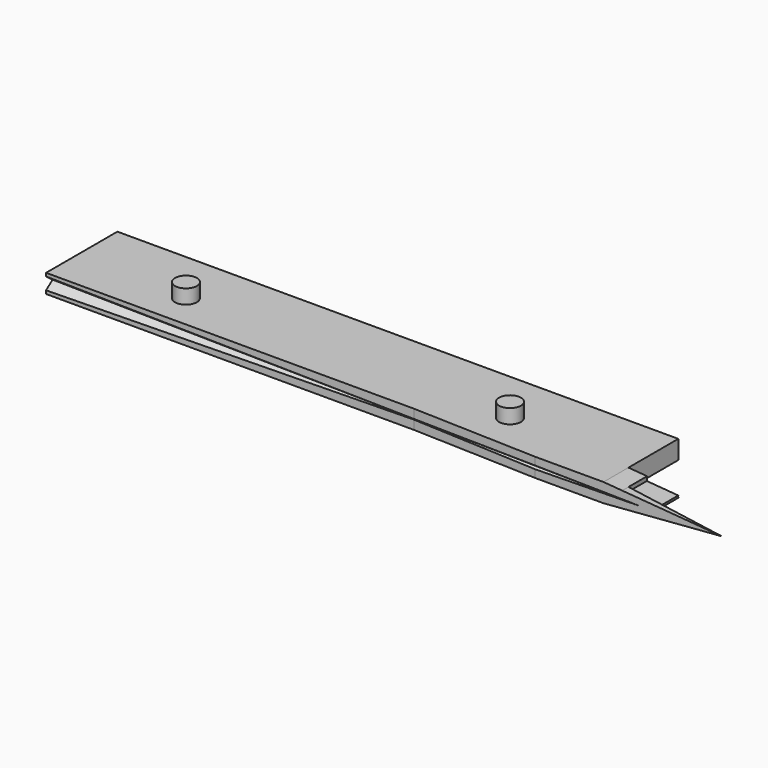
from build123d import *

# Parameters (mm, degrees)
F1_DEPTH  = 1.5
F3_DEPTH  = 25
F4_DEPTH  = 5
F6_W      = 90
F6_H      = 3
F7_DEPTH  = 5
F5_R      = 1.75
F8_DEPTH  = 3.8
F9_W      = 16.7752551286
F9_H      = 3
F9_W_2    = 2.4494897428
F9_W_3    = 49.5505102572
F9_W_4    = 18.7752551286
F10_DEPTH = 10
F15_DEPTH = 5.301


# Not quite as in the source:
# - ends of sketch curves that miss each other by under 0.0002 mm in the source are joined


with BuildPart() as f1:
    # F0 (on Front) → F1 (new body)
    with BuildSketch(Plane.XZ):
        Polygon((0, -0.8), (0, -1.5), (3, -1.2631578947), (2.9450791466, -0.5674937516), align=None)
        Polygon((2.9450791466, -0.5674937516), (3, -1.2631578947), (19, 0), (10.1333333333, 0), (8, -0.1684210526), align=None)
        Polygon((0, 0), (0, -0.8), (2.9450791466, -0.5674937516), (8, -0.1684210526), (7.9867036011, 0), align=None)
        Polygon((10.1333333333, 0), (19, 0), (3, 1.2631578947), (2.9450791466, 0.5674937516), (8, 0.1684210526), align=None)
        Polygon((0, 0.8), (0, 0), (7.9867036011, 0), (8, 0.1684210526), (2.9450791466, 0.5674937516), align=None)
        Polygon((2.9450791466, 0.5674937516), (3, 1.2631578947), (0, 1.5), (0, 0.8), align=None)
        Polygon((8, -0.1684210526), (10.1333333333, 0), (7.9867036011, 0), align=None)
        Polygon((7.9867036011, 0), (10.1333333333, 0), (8, 0.1684210526), align=None)
    extrude(amount=-F1_DEPTH)

    # F2 (on face) → F3 (cut)
    with BuildSketch(Plane(origin=(0.117687543, 0, 1.4907088782), x_dir=(0.9968981487, 0, -0.0787024854), z_dir=(0.0787024854, 0, 0.9968981487))):
        Polygon((18.9410648244, 1.5), (-0.1180537281, 1.5), (18.9410648244, 0), align=None)
    extrude(amount=-F3_DEPTH, mode=Mode.SUBTRACT)

    # F0 (on Front) → F4 (join)
    with BuildSketch(Plane.XZ):
        Polygon((0, 0.8), (0, 0), (7.9867036011, 0), (8, 0.1684210526), (2.9450791466, 0.5674937516), align=None)
        Polygon((0, 0), (0, -0.8), (2.9450791466, -0.5674937516), (8, -0.1684210526), (7.9867036011, 0), align=None)
        Polygon((0, -0.8), (0, -1.5), (3, -1.2631578947), (2.9450791466, -0.5674937516), align=None)
        Polygon((2.9450791466, 0.5674937516), (3, 1.2631578947), (0, 1.5), (0, 0.8), align=None)
    extrude(amount=-F4_DEPTH)

    # F6 (on face) → F7 (join, through all)
    with BuildSketch(Plane.XZ):
        with Locations((-45, 0)):
            Rectangle(F6_W, F6_H)
    extrude(amount=-F7_DEPTH)

    # F5 (on Top) → F8 (join, symmetric)
    with BuildSketch(Plane.XY):
        with Locations((-20, 6.25)):
            Circle(F5_R)
        with Locations((-72, 6.25)):
            Circle(F5_R)
    extrude(amount=F8_DEPTH, both=True)

    # F9 (on face) → F10 (join)
    with BuildSketch(Plane(origin=(0, 5, 0), x_dir=(-1, 0, 0), z_dir=(0, 1, 0))):
        with Locations((81.6123724357, 0)):
            Rectangle(F9_W, F9_H)
        with Locations((72, 0)):
            Rectangle(F9_W_2, F9_H)
        with Locations((46, 0)):
            Rectangle(F9_W_3, F9_H)
        with Locations((20, 0)):
            Rectangle(F9_W_2, F9_H)
        with Locations((9.3876275643, 0)):
            Rectangle(F9_W_4, F9_H)
    extrude(amount=F10_DEPTH)

    # F13: sweep along a path in F11
    with BuildLine(Plane.XY) as f13_path:
        Line((-90, 2), (6, 0))
    # F12 (on face) → F13 (sweep, cut)
    with BuildSketch(Plane(origin=(-90, 0, 0), x_dir=(0, -1, 0), z_dir=(-1, 0, 0))):
        Polygon((-2, 0), (0, -1.5), (0, 1.5), align=None)
    sweep(path=f13_path.line, mode=Mode.SUBTRACT)

    # F14 (on face) → F15 (cut, through all)
    with BuildSketch(Plane.XY.offset(1.5)):
        Polygon((-90, 0.7), (-90, 0), (-10.954622702, 0), (-31, 0.7), align=None)
    extrude(amount=-F15_DEPTH, mode=Mode.SUBTRACT)


solid = f1.part
